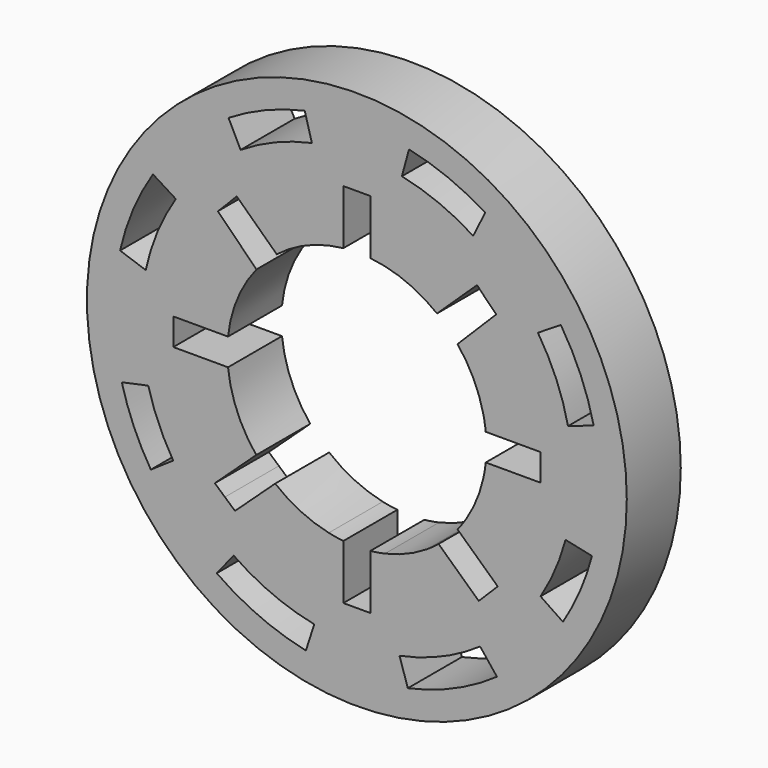
from build123d import *

# Parameters (mm, degrees)
F0_R     = 12.7
F1_DEPTH = 3.175


# Not quite as in the source:
# - ends of sketch curves that miss each other by under 0.0002 mm in the source are joined


with BuildPart() as f1:
    # F0 (on Front) → F1 (new body)
    with BuildSketch(Plane.XZ):
        Circle(F0_R)
        with BuildLine():
            ThreePointArc((11.1424209807, 2.5478137078), (11.3578777025, 1.2819961371), (11.43, 0))
            ThreePointArc((11.43, 0), (11.3372924765, -1.4528245947), (11.0606737878, -2.8820817755))
            ThreePointArc((11.0606737878, -2.8820817755), (10.498054115, -4.5205928591), (9.694266327, -6.0552539485))
            ThreePointArc((9.694266327, -6.0552539485), (8.3067678362, -7.8512742988), (6.5917644701, -9.3377481852))
            ThreePointArc((6.5917644701, -9.3377481852), (4.5881966593, -10.4686843212), (2.3987302505, -11.1754638913))
            ThreePointArc((2.3987302505, -11.1754638913), (0, -11.43), (-2.3987302505, -11.1754638913))
            ThreePointArc((-2.3987302505, -11.1754638913), (-4.5881966593, -10.4686843212), (-6.5917644701, -9.3377481852))
            ThreePointArc((-6.5917644701, -9.3377481852), (-8.3067678362, -7.8512742988), (-9.694266327, -6.0552539485))
            ThreePointArc((-9.694266327, -6.0552539485), (-10.498054115, -4.5205928591), (-11.0606737878, -2.8820817755))
            ThreePointArc((-11.0606737878, -2.8820817755), (-11.4287048944, -0.1720593972), (-11.1424209807, 2.5478137078))
            ThreePointArc((-11.1424209807, 2.5478137078), (-10.5290706386, 4.4478726922), (-9.5944423354, 6.2122118663))
            ThreePointArc((-9.5944423354, 6.2122118663), (-8.0092161617, 8.1545911286), (-6.0386388222, 9.7046247313))
            ThreePointArc((-6.0386388222, 9.7046247313), (-4.3084616277, 10.5868814295), (-2.4538934823, 11.1634809436))
            ThreePointArc((-2.4538934823, 11.1634809436), (0, 11.43), (2.4538934823, 11.1634809436))
            ThreePointArc((2.4538934823, 11.1634809436), (4.3084616277, 10.5868814295), (6.0386388222, 9.7046247313))
            ThreePointArc((6.0386388222, 9.7046247313), (8.0092161617, 8.1545911286), (9.5944423354, 6.2122118663))
            ThreePointArc((9.5944423354, 6.2122118663), (10.5290706386, 4.4478726922), (11.1424209807, 2.5478137078))
        make_face(mode=Mode.SUBTRACT)
        with BuildLine():
            ThreePointArc((10.16, 0), (10.10329164, 1.0719599045), (9.933799599, 2.1319534531))
            ThreePointArc((9.933799599, 2.1319534531), (9.3818599064, 3.8995262145), (8.5182733268, 5.5375644041))
            ThreePointArc((8.5182733268, 5.5375644041), (7.1564472405, 7.2118557178), (5.4717026611, 8.5607283562))
            ThreePointArc((5.4717026611, 8.5607283562), (3.8560932614, 9.3997949318), (2.1166776906, 9.9370657417))
            ThreePointArc((2.1166776906, 9.9370657417), (0, 10.16), (-2.1166776906, 9.9370657417))
            ThreePointArc((-2.1166776906, 9.9370657417), (-3.8560932614, 9.3997949318), (-5.4717026611, 8.5607283562))
            ThreePointArc((-5.4717026611, 8.5607283562), (-7.1564472405, 7.2118557178), (-8.5182733268, 5.5375644041))
            ThreePointArc((-8.5182733268, 5.5375644041), (-9.3818599064, 3.8995262145), (-9.933799599, 2.1319534531))
            ThreePointArc((-9.933799599, 2.1319534531), (-10.1569477884, -0.2490213305), (-9.817387512, -2.6162))
            ThreePointArc((-9.817387512, -2.6162), (-9.3301072422, -4.0217780707), (-8.6427953563, -5.3411317555))
            ThreePointArc((-8.6427953563, -5.3411317555), (-7.3747174058, -6.9885007824), (-5.7978750028, -8.343275463))
            ThreePointArc((-5.7978750028, -8.343275463), (-3.9840291181, -9.3462886744), (-2.0043747759, -9.9603253841))
            ThreePointArc((-2.0043747759, -9.9603253841), (0, -10.16), (2.0043747759, -9.9603253841))
            ThreePointArc((2.0043747759, -9.9603253841), (3.9840291181, -9.3462886744), (5.7978750028, -8.343275463))
            ThreePointArc((5.7978750028, -8.343275463), (7.3747174058, -6.9885007824), (8.6427953563, -5.3411317555))
            ThreePointArc((8.6427953563, -5.3411317555), (9.3301072422, -4.0217780707), (9.817387512, -2.6162))
            ThreePointArc((9.817387512, -2.6162), (10.0739827556, -1.3192692823), (10.16, 0))
        make_face()
        with BuildLine():
            ThreePointArc((4.7360858752, 3.8380602631), (5.4892872515, 2.6512150932), (5.9506155559, 1.323401113))
            Line((5.9506155559, 1.323401113), (8.636, 1.323401113))
            Line((8.636, 1.323401113), (8.636, 0.635))
            Line((8.636, 0.635), (8.636, 0))
            Line((8.636, 0), (8.636, -0.635))
            Line((8.636, -0.635), (8.636, -1.323401113))
            Line((8.636, -1.323401113), (5.9506155559, -1.323401113))
            ThreePointArc((5.9506155559, -1.323401113), (5.6312135784, -2.3346626382), (5.1413854537, -3.2752666482))
            Line((5.1413854537, -3.2752666482), (7.0945855376, -5.080295188))
            Line((7.0945855376, -5.080295188), (6.6273668913, -5.5858669721))
            Line((6.6273668913, -5.5858669721), (5.7343752763, -6.4777944262))
            Line((5.7343752763, -6.4777944262), (5.2671687856, -6.9833774435))
            Line((5.2671687856, -6.9833774435), (3.2744427263, -5.1419102319))
            ThreePointArc((3.2744427263, -5.1419102319), (2.3342114446, -5.631400619), (1.323401113, -5.9506155559))
            Line((1.323401113, -5.9506155559), (1.323401113, -8.636))
            Line((1.323401113, -8.636), (0.635, -8.636))
            Line((0.635, -8.636), (0, -8.636))
            Line((0, -8.636), (-0.635, -8.636))
            Line((-0.635, -8.636), (-1.323401113, -8.636))
            Line((-1.323401113, -8.636), (-1.323401113, -5.9506155559))
            ThreePointArc((-1.323401113, -5.9506155559), (-2.6547777921, -5.4875651135), (-3.8442056919, -4.7310990899))
            Line((-3.8442056919, -4.7310990899), (-5.7343752763, -6.4777944262))
            Line((-5.7343752763, -6.4777944262), (-6.2091766623, -6.0579455764))
            Line((-6.2091766623, -6.0579455764), (-6.6839780483, -5.6380967267))
            Line((-6.6839780483, -5.6380967267), (-4.7360858752, -3.8380602631))
            ThreePointArc((-4.7360858752, -3.8380602631), (-5.6319696302, -2.3328382037), (-6.0628368772, -0.635))
            Line((-6.0628368772, -0.635), (-8.636, -0.635))
            Line((-8.636, -0.635), (-8.636, 0))
            Line((-8.636, 0), (-8.636, 0.635))
            Line((-8.636, 0.635), (-6.0628368772, 0.635))
            ThreePointArc((-6.0628368772, 0.635), (-5.6281633501, 2.3420062564), (-4.7235609165, 3.8534644501))
            Line((-4.7235609165, 3.8534644501), (-6.5416064283, 5.671509962))
            Line((-6.5416064283, 5.671509962), (-6.0925936223, 6.120522768))
            Line((-6.0925936223, 6.120522768), (-5.6552171182, 6.5808778416))
            Line((-5.6552171182, 6.5808778416), (-3.7703908438, 4.7901324496))
            ThreePointArc((-3.7703908438, 4.7901324496), (-2.2927737049, 5.6483984224), (-0.635, 6.0628368772))
            Line((-0.635, 6.0628368772), (-0.635, 8.636))
            Line((-0.635, 8.636), (0, 8.636))
            Line((0, 8.636), (0.635, 8.636))
            Line((0.635, 8.636), (0.635, 6.0628368772))
            ThreePointArc((0.635, 6.0628368772), (2.2927737049, 5.6483984224), (3.7703908438, 4.7901324496))
            Line((3.7703908438, 4.7901324496), (5.6552171182, 6.5808778416))
            Line((5.6552171182, 6.5808778416), (6.0925936223, 6.120522768))
            Line((6.0925936223, 6.120522768), (6.1065741623, 6.1065741623))
            Line((6.1065741623, 6.1065741623), (6.5416223955, 5.6715259292))
            Line((6.5416223955, 5.6715259292), (6.5555869684, 5.6575613563))
            Line((6.5555869684, 5.6575613563), (4.7360858752, 3.8380602631))
        make_face(mode=Mode.SUBTRACT)
        with BuildLine():
            ThreePointArc((11.0606737878, -2.8820817755), (11.3372924765, -1.4528245947), (11.43, 0))
            ThreePointArc((11.43, 0), (11.3578777025, 1.2819961371), (11.1424209807, 2.5478137078))
            Line((11.1424209807, 2.5478137078), (9.933799599, 2.1319534531))
            ThreePointArc((9.933799599, 2.1319534531), (10.10329164, 1.0719599045), (10.16, 0))
            ThreePointArc((10.16, 0), (10.0739827556, -1.3192692823), (9.817387512, -2.6162))
            Line((9.817387512, -2.6162), (11.0606737878, -2.8820817755))
        make_face()
        with BuildLine():
            Line((-9.933799599, 2.1319534531), (-11.1424209807, 2.5478137078))
            ThreePointArc((-11.1424209807, 2.5478137078), (-11.4287048944, -0.1720593972), (-11.0606737878, -2.8820817755))
            Line((-11.0606737878, -2.8820817755), (-9.817387512, -2.6162))
            ThreePointArc((-9.817387512, -2.6162), (-10.1569477884, -0.2490213305), (-9.933799599, 2.1319534531))
        make_face()
        with BuildLine():
            Line((-5.4717026611, 8.5607283562), (-6.0386388222, 9.7046247313))
            ThreePointArc((-6.0386388222, 9.7046247313), (-8.0092161617, 8.1545911286), (-9.5944423354, 6.2122118663))
            Line((-9.5944423354, 6.2122118663), (-8.5182733268, 5.5375644041))
            ThreePointArc((-8.5182733268, 5.5375644041), (-7.1564472405, 7.2118557178), (-5.4717026611, 8.5607283562))
        make_face()
        with BuildLine():
            Line((8.5182733268, 5.5375644041), (9.5944423354, 6.2122118663))
            ThreePointArc((9.5944423354, 6.2122118663), (8.0092161617, 8.1545911286), (6.0386388222, 9.7046247313))
            Line((6.0386388222, 9.7046247313), (5.4717026611, 8.5607283562))
            ThreePointArc((5.4717026611, 8.5607283562), (7.1564472405, 7.2118557178), (8.5182733268, 5.5375644041))
        make_face()
        with BuildLine():
            Line((2.1166776906, 9.9370657417), (2.4538934823, 11.1634809436))
            ThreePointArc((2.4538934823, 11.1634809436), (0, 11.43), (-2.4538934823, 11.1634809436))
            Line((-2.4538934823, 11.1634809436), (-2.1166776906, 9.9370657417))
            ThreePointArc((-2.1166776906, 9.9370657417), (0, 10.16), (2.1166776906, 9.9370657417))
        make_face()
        with BuildLine():
            ThreePointArc((-2.3987302505, -11.1754638913), (0, -11.43), (2.3987302505, -11.1754638913))
            Line((2.3987302505, -11.1754638913), (2.0043747759, -9.9603253841))
            ThreePointArc((2.0043747759, -9.9603253841), (0, -10.16), (-2.0043747759, -9.9603253841))
            Line((-2.0043747759, -9.9603253841), (-2.3987302505, -11.1754638913))
        make_face()
        with BuildLine():
            ThreePointArc((6.5917644701, -9.3377481852), (8.3067678362, -7.8512742988), (9.694266327, -6.0552539485))
            Line((9.694266327, -6.0552539485), (8.6427953563, -5.3411317555))
            ThreePointArc((8.6427953563, -5.3411317555), (7.3747174058, -6.9885007824), (5.7978750028, -8.343275463))
            Line((5.7978750028, -8.343275463), (6.5917644701, -9.3377481852))
        make_face()
        with BuildLine():
            ThreePointArc((-9.694266327, -6.0552539485), (-8.3067678362, -7.8512742988), (-6.5917644701, -9.3377481852))
            Line((-6.5917644701, -9.3377481852), (-5.7978750028, -8.343275463))
            ThreePointArc((-5.7978750028, -8.343275463), (-7.3747174058, -6.9885007824), (-8.6427953563, -5.3411317555))
            Line((-8.6427953563, -5.3411317555), (-9.694266327, -6.0552539485))
        make_face()
        with BuildLine():
            Line((5.7343752763, -6.4777944262), (3.8442056919, -4.7310990899))
            ThreePointArc((3.8442056919, -4.7310990899), (3.565246173, -4.9447179623), (3.2744427263, -5.1419102319))
            Line((3.2744427263, -5.1419102319), (5.2671687856, -6.9833774435))
            Line((5.2671687856, -6.9833774435), (5.7343752763, -6.4777944262))
        make_face()
        with BuildLine():
            Line((1.323401113, -8.636), (1.323401113, -5.9506155559))
            ThreePointArc((1.323401113, -5.9506155559), (0.9808068801, -6.0165799142), (0.635, -6.0628368772))
            Line((0.635, -6.0628368772), (0.635, -8.636))
            Line((0.635, -8.636), (1.323401113, -8.636))
        make_face()
        with BuildLine():
            Line((-0.635, -8.636), (-0.635, -6.0628368772))
            ThreePointArc((-0.635, -6.0628368772), (-0.9808068801, -6.0165799142), (-1.323401113, -5.9506155559))
            Line((-1.323401113, -5.9506155559), (-1.323401113, -8.636))
            Line((-1.323401113, -8.636), (-0.635, -8.636))
        make_face()
        with BuildLine():
            Line((8.636, -0.635), (6.0628368772, -0.635))
            ThreePointArc((6.0628368772, -0.635), (6.0165799142, -0.9808068801), (5.9506155559, -1.323401113))
            Line((5.9506155559, -1.323401113), (8.636, -1.323401113))
            Line((8.636, -1.323401113), (8.636, -0.635))
        make_face()
        with BuildLine():
            ThreePointArc((5.9506155559, 1.323401113), (6.0165799142, 0.9808068801), (6.0628368772, 0.635))
            Line((6.0628368772, 0.635), (8.636, 0.635))
            Line((8.636, 0.635), (8.636, 1.323401113))
            Line((8.636, 1.323401113), (5.9506155559, 1.323401113))
        make_face()
        with BuildLine():
            Line((7.0945855376, -5.080295188), (5.1413854537, -3.2752666482))
            ThreePointArc((5.1413854537, -3.2752666482), (4.9467458118, -3.5624320167), (4.7360858752, -3.8380602631))
            Line((4.7360858752, -3.8380602631), (6.6273668913, -5.5858669721))
            Line((6.6273668913, -5.5858669721), (7.0945855376, -5.080295188))
        make_face()
    extrude(amount=F1_DEPTH)


solid = f1.part
